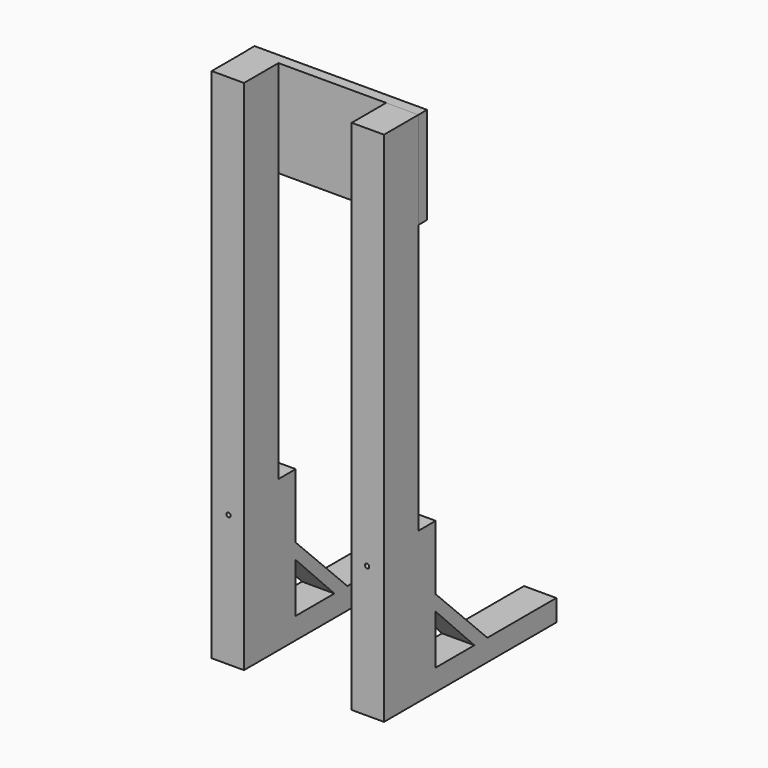
from build123d import *

# Parameters (mm, degrees)
F1_DEPTH = 9.525
F5_D     = 2.54
F5_2_D   = 2.54
F6_W     = 82.682737267
F6_H     = 19.1611907959
F6_H_2   = 18.3808207512
F6_H_3   = 19.627019763
F6_W_2   = 19.05
F7_DEPTH = 6.35


with BuildPart() as f1:
    # F0 (on Right) → F1 (new body, symmetric)
    with BuildSketch(Plane.YZ):
        Polygon((-25.4, 0), (0, 0), (0, 12.7), (0, 88.9), (0, 304.8), (-25.4, 304.8), align=None)
        Polygon((0, 88.9), (0, 12.7), (12.7, 12.7), (12.7, 41.7682752013), (12.7, 50.8), (12.7, 88.9), align=None)
        Polygon((41.2119701505, 12.7), (50.8, 12.7), (12.7, 50.8), (12.7, 41.7682752013), align=None)
        Polygon((0, 12.7), (0, 0), (101.6, 0), (101.6, 12.7), (50.8, 12.7), (41.2119701505, 12.7), (12.7, 12.7), align=None)
    extrude(amount=F1_DEPTH, both=True)


with BuildPart() as f3_1:
    # F3: instance of F1
    add(f1.part.mirror(Plane(origin=(-41.275, -1.6869500415, 120.8741886465), x_dir=(0, 1, 0), z_dir=(-1, 0, 0))))

    # F5#2 (through all)
    with Locations(Plane(origin=(0, 12.7, 0), x_dir=(-1, 0, 0), z_dir=(0, 1, 0))):
        with Locations((0.4395503283, 77.6355564594), (82.1104496717, 77.6355564594)):
            Hole(F5_2_D / 2)

    # F6 (on face) → F7 (join)
    with BuildSketch(Plane(origin=(0, 0, 0), x_dir=(-1, 0, 0), z_dir=(0, 1, 0))):
        with Locations((50.8663686335, 295.2194046021)):
            Rectangle(F6_W, F6_H)
        with Locations((50.8663686335, 276.4483988285)):
            Rectangle(F6_W, F6_H_2)
        with Locations((50.8663686335, 257.4444785714)):
            Rectangle(F6_W, F6_H_3)
        with Locations((0, 295.2194046021)):
            Rectangle(F6_W_2, F6_H)
        with Locations((0, 276.4483988285)):
            Rectangle(F6_W_2, F6_H_2)
        with Locations((0, 257.4444785714)):
            Rectangle(F6_W_2, F6_H_3)
    extrude(amount=F7_DEPTH)


with BuildPart() as f1_1:
    add(f1.part)

    # F5 (through all)
    with Locations(Plane(origin=(0, 12.7, 0), x_dir=(-1, 0, 0), z_dir=(0, 1, 0))):
        with Locations((0.4395503283, 77.6355564594), (82.1104496717, 77.6355564594)):
            Hole(F5_D / 2)


solid = Compound([f3_1.part, f1_1.part])
